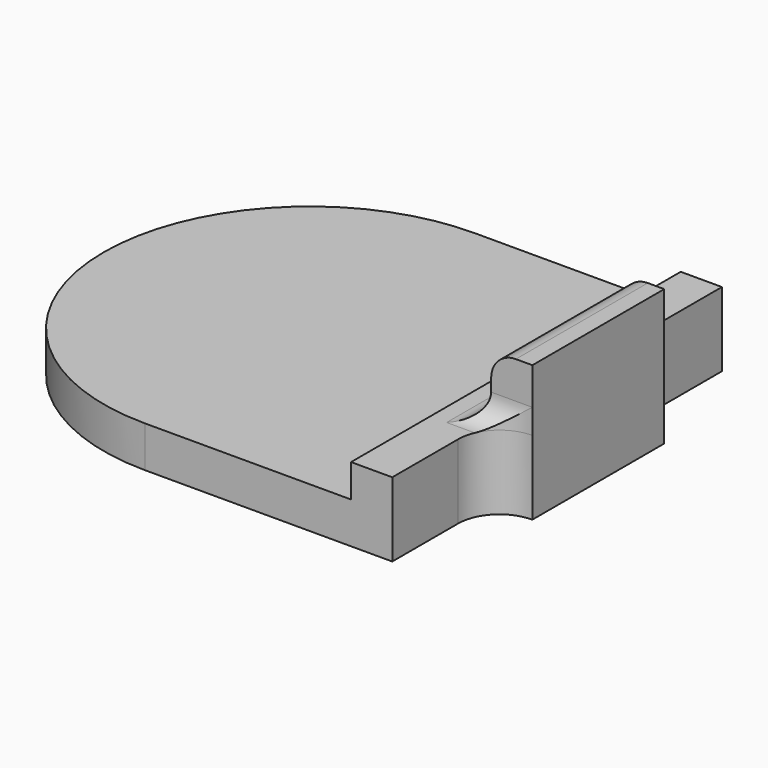
from build123d import *

# Parameters (mm, degrees)
F1_DEPTH     = 5
F2_W         = 5
F2_H         = 50
F3_DEPTH     = 4
F4_W         = 5
F4_H         = 20
F5_DEPTH     = 11.5
F6_T1_DEPTH  = 9
F7_T1_DEPTH  = 20
F7_T6_DEPTH  = 5
F7_S7_R      = 5.0000000001
F7_T8_DEPTH  = 5
F7_T12_DEPTH = 5
F7_S13_R     = 5.0000000001
F7_T14_DEPTH = 5
F7_T19_DEPTH = 12.5
F7_T24_DEPTH = 27.5
F7_T31_DEPTH = 27.5
F7_T35_DEPTH = 12.5
F7_T39_DEPTH = 35


# Not quite as in the source:
# - a fillet or chamfer that OpenCascade refuses, or shapes differently, is made with other operations: its cross-section is extruded or revolved along the edge and cut away or added


with BuildPart() as f1:
    # F0 (on Top) → F1 (new body)
    with BuildSketch(Plane.XY):
        with BuildLine():
            Line((30, 25), (0, 25))
            ThreePointArc((0, 25), (-25, 0), (0, -25))
            Line((0, -25), (30, -25))
            Line((30, -25), (30, -10))
            Line((30, -10), (35, -10))
            Line((35, -10), (35, 10))
            Line((35, 10), (30, 10))
            Line((30, 10), (30, 25))
        make_face()
    extrude(amount=F1_DEPTH)

    # F2 (on face) → F3 (join)
    with BuildSketch(Plane.XY.offset(5)):
        with Locations((27.5, 0)):
            Rectangle(F2_W, F2_H)
    extrude(amount=F3_DEPTH)

    # F4 (on face) → F5 (join)
    with BuildSketch(Plane.XY.offset(5)):
        with Locations((32.5, 0)):
            Rectangle(F4_W, F4_H)
    extrude(amount=F5_DEPTH)

    # F6: fillet of radius 5 on 3 edges, made by hand

    # F6_s2 → F6_t1 (join)
    with BuildSketch(Plane.XY):
        with BuildLine():
            ThreePointArc((30, -15), (31.4644660941, -11.4644660941), (35, -10))
            Line((35, -10), (30, -10))
            Line((30, -10), (30, -15))
        make_face()
        with BuildLine():
            ThreePointArc((30, 15), (31.4644660941, 11.4644660941), (35, 10))
            Line((35, 10), (30, 10))
            Line((30, 10), (30, 15))
        make_face()
    extrude(amount=F6_T1_DEPTH)

    # F7: fillet of radius 3 on 4 edges, made by hand

    # F7_s2 → F7_t1 (join)
    with BuildSketch(Plane.XZ.offset(-10)):
        with BuildLine():
            ThreePointArc((27, 9), (29.1213203436, 9.8786796564), (30, 12))
            Line((30, 12), (30, 9))
            Line((30, 9), (27, 9))
        make_face()
    extrude(amount=F7_T1_DEPTH)


with BuildPart() as f7_tool4:
    # F7_s5 → F7_t6 (new body)
    with BuildSketch(Plane.YZ.offset(35)):
        with BuildLine():
            ThreePointArc((-13, 9), (-10.8786796564, 9.8786796564), (-10, 12))
            Line((-10, 12), (-10, 9))
            Line((-10, 9), (-13, 9))
        make_face()
    extrude(amount=-F7_T6_DEPTH)

    # F7_s7 → F7_t8 (cut, symmetric)
    with BuildSketch(Plane.XY.offset(10.5)):
        with Locations((35.0000000001, -15.0000000001)):
            Circle(F7_S7_R)
    extrude(amount=F7_T8_DEPTH, both=True, mode=Mode.SUBTRACT)


with BuildPart() as f1_1:
    add(f1.part)

    # F7_t3: union F7_tool4
    add(f7_tool4.part)


with BuildPart() as f7_tool10:
    # F7_s11 → F7_t12 (new body)
    with BuildSketch(Plane.YZ.offset(35)):
        with BuildLine():
            ThreePointArc((13, 9), (10.8786796564, 9.8786796564), (10, 12))
            Line((10, 12), (10, 9))
            Line((10, 9), (13, 9))
        make_face()
    extrude(amount=-F7_T12_DEPTH)

    # F7_s13 → F7_t14 (cut, symmetric)
    with BuildSketch(Plane.XY.offset(10.5)):
        with Locations((35.0000000001, 15.0000000001)):
            Circle(F7_S13_R)
    extrude(amount=F7_T14_DEPTH, both=True, mode=Mode.SUBTRACT)


with BuildPart() as f1_2:
    add(f1_1.part)

    # F7_t9: union F7_tool10
    add(f7_tool10.part)


with BuildPart() as f7_tool17:
    # F7_s18 → F7_t19 (new body)
    with BuildSketch(Plane.YZ.offset(35)):
        with BuildLine():
            ThreePointArc((-13, 9), (-10.8786796564, 9.8786796564), (-10, 12))
            Line((-10, 12), (-10, 9))
            Line((-10, 9), (-13, 9))
        make_face()
    extrude(amount=-F7_T19_DEPTH)

    split(bisect_by=Plane.YZ.offset(25), keep=Keep.TOP)

    split(bisect_by=Plane.YZ.offset(30), keep=Keep.BOTTOM)


with BuildPart() as f7_tool22:
    # F7_s23 → F7_t24 (new body)
    with BuildSketch(Plane.XZ.offset(17.5)):
        with BuildLine():
            ThreePointArc((27, 9), (29.1213203436, 9.8786796564), (30, 12))
            Line((30, 12), (30, 9))
            Line((30, 9), (27, 9))
        make_face()
    extrude(amount=-F7_T24_DEPTH)

    split(bisect_by=Plane.XZ.offset(10), keep=Keep.TOP)


with BuildPart() as f7_tool17_1:
    add(f7_tool17.part)

    # F7_t26: intersect F7_tool22
    add(f7_tool22.part, mode=Mode.INTERSECT)


with BuildPart() as f1_3:
    add(f1_2.part)

    # F7_t15: union F7_tool17
    add(f7_tool17_1.part)


with BuildPart() as f7_tool29:
    # F7_s30 → F7_t31 (new body)
    with BuildSketch(Plane.XZ.offset(10)):
        with BuildLine():
            ThreePointArc((27, 9), (29.1213203436, 9.8786796564), (30, 12))
            Line((30, 12), (30, 9))
            Line((30, 9), (27, 9))
        make_face()
    extrude(amount=-F7_T31_DEPTH)

    split(bisect_by=Plane.XZ.offset(-10), keep=Keep.BOTTOM)


with BuildPart() as f7_tool33:
    # F7_s34 → F7_t35 (new body)
    with BuildSketch(Plane.YZ.offset(35)):
        with BuildLine():
            ThreePointArc((13, 9), (10.8786796564, 9.8786796564), (10, 12))
            Line((10, 12), (10, 9))
            Line((10, 9), (13, 9))
        make_face()
    extrude(amount=-F7_T35_DEPTH)

    split(bisect_by=Plane.YZ.offset(25), keep=Keep.TOP)

    split(bisect_by=Plane.YZ.offset(30), keep=Keep.BOTTOM)


with BuildPart() as f7_tool29_1:
    add(f7_tool29.part)

    # F7_t38: intersect F7_tool33
    add(f7_tool33.part, mode=Mode.INTERSECT)


with BuildPart() as f1_4:
    add(f1_3.part)

    # F7_t27: union F7_tool29
    add(f7_tool29_1.part)

    # F7_s40 → F7_t39 (cut)
    with BuildSketch(Plane.XZ.offset(-17.5)):
        with BuildLine():
            ThreePointArc((30, 13.5), (30.8786796564, 15.6213203436), (33, 16.5))
            Line((33, 16.5), (30, 16.5))
            Line((30, 16.5), (30, 13.5))
        make_face()
    extrude(amount=F7_T39_DEPTH, mode=Mode.SUBTRACT)


solid = f1_4.part
